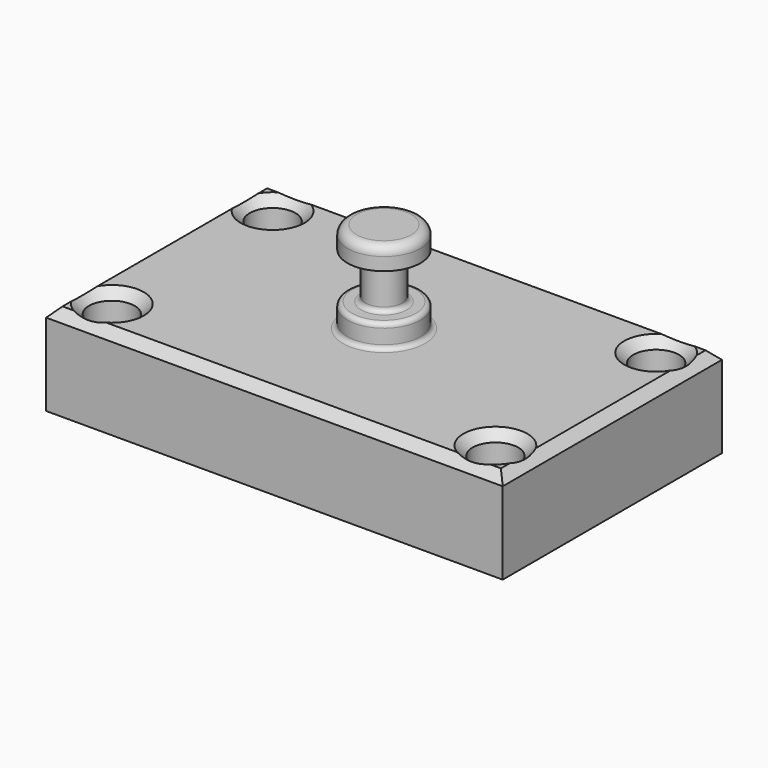
from build123d import *

# Parameters (mm, degrees)
F0_W         = 127
F0_H         = 76.2
F1_DEPTH     = 25.4
F2_R         = 6.35
F3_DEPTH     = 25.401
F4_W         = 10.16
F4_H         = 25.4
F6_W         = 15.24
F6_H         = 12.7
F8_R         = 2.54
F9_R         = 1.27
F10_T1_DEPTH = 140.0641495789
F10_T3_DEPTH = 89.2641495789


# Not quite as in the source:
# - a fillet or chamfer that OpenCascade refuses, or shapes differently, is made with other operations: its cross-section is extruded or revolved along the edge and cut away or added


with BuildPart() as f1:
    # F0 (on Top) → F1 (new body)
    with BuildSketch(Plane.XY):
        Rectangle(F0_W, F0_H)
    extrude(amount=F1_DEPTH)

    # F2 (on face) → F3 (cut, through all)
    with BuildSketch(Plane.XY.offset(25.4)):
        with Locations((53.34, 27.94)):
            Circle(F2_R)
        with Locations((53.34, -27.94)):
            Circle(F2_R)
        with Locations((-53.34, 27.94)):
            Circle(F2_R)
        with Locations((-53.34, -27.94)):
            Circle(F2_R)
    extrude(amount=-F3_DEPTH, mode=Mode.SUBTRACT)

    # F4 (on Front) → F5 (revolve)
    with BuildSketch(Plane.XZ):
        with Locations((5.08, 38.1)):
            Rectangle(F4_W, F4_H)
    revolve(axis=Axis((0, 0, 38.1), (0, 0, -1)))

    # F6 (on Front) → F7 (revolve, cut)
    with BuildSketch(Plane.XZ):
        with Locations((12.7, 38.3218890125)):
            Rectangle(F6_W, F6_H)
    revolve(axis=Axis((0, 0, 25.4), (0, 0, 1)), mode=Mode.SUBTRACT)

    # F8
    f8_edges = [f1.edges().sort_by_distance(p)[0] for p in [
        (-10.16, 0, 50.8),
    ]]
    fillet(f8_edges, radius=F8_R)

    # F9
    f9_edges = [f1.edges().sort_by_distance(p)[0] for p in [
        (-10.16, 0, 31.971889),
        (-5.08, 0, 31.971889),
        (-10.16, 0, 25.4),
    ]]
    fillet(f9_edges, radius=F9_R)

    # F10: chamfer of 2.54 on 9 edges, made by hand

    # F10_s2 → F10_t1 (cut)
    with BuildSketch(Plane.YZ.offset(-70.0320747894)):
        Polygon((35.56, 25.4), (38.1, 22.86), (38.1, 25.4), align=None)
        Polygon((-35.56, 25.4), (-38.1, 22.86), (-38.1, 25.4), align=None)
    extrude(amount=F10_T1_DEPTH, mode=Mode.SUBTRACT)

    # F10_s4 → F10_t3 (cut)
    with BuildSketch(Plane.XZ.offset(-44.6320747894)):
        Polygon((60.96, 25.4), (63.5, 22.86), (63.5, 25.4), align=None)
        Polygon((-60.96, 25.4), (-63.5, 22.86), (-63.5, 25.4), align=None)
    extrude(amount=F10_T3_DEPTH, mode=Mode.SUBTRACT)

    # F10_s5 → F10_t6 (revolve, cut)
    with BuildSketch(Plane.XZ.offset(27.94)):
        Polygon((-44.45, 25.4), (-46.99, 22.86), (-46.99, 25.4), align=None)
    revolve(axis=Axis((-53.34, -27.94, 25.4), (0, 0, 1)), mode=Mode.SUBTRACT)

    # F10_s7 → F10_t8 (revolve, cut)
    with BuildSketch(Plane.XZ.offset(27.94)):
        Polygon((62.23, 25.4), (59.69, 22.86), (59.69, 25.4), align=None)
    revolve(axis=Axis((53.34, -27.94, 25.4), (0, 0, 1)), mode=Mode.SUBTRACT)

    # F10_s9 → F10_t10 (revolve, cut)
    with BuildSketch(Plane.XZ.offset(-27.94)):
        Polygon((-44.45, 25.4), (-46.99, 22.86), (-46.99, 25.4), align=None)
    revolve(axis=Axis((-53.34, 27.94, 25.4), (0, 0, 1)), mode=Mode.SUBTRACT)

    # F10_s11 → F10_t12 (revolve, cut)
    with BuildSketch(Plane.XZ.offset(-27.94)):
        Polygon((62.23, 25.4), (59.69, 22.86), (59.69, 25.4), align=None)
    revolve(axis=Axis((53.34, 27.94, 25.4), (0, 0, 1)), mode=Mode.SUBTRACT)


solid = f1.part
